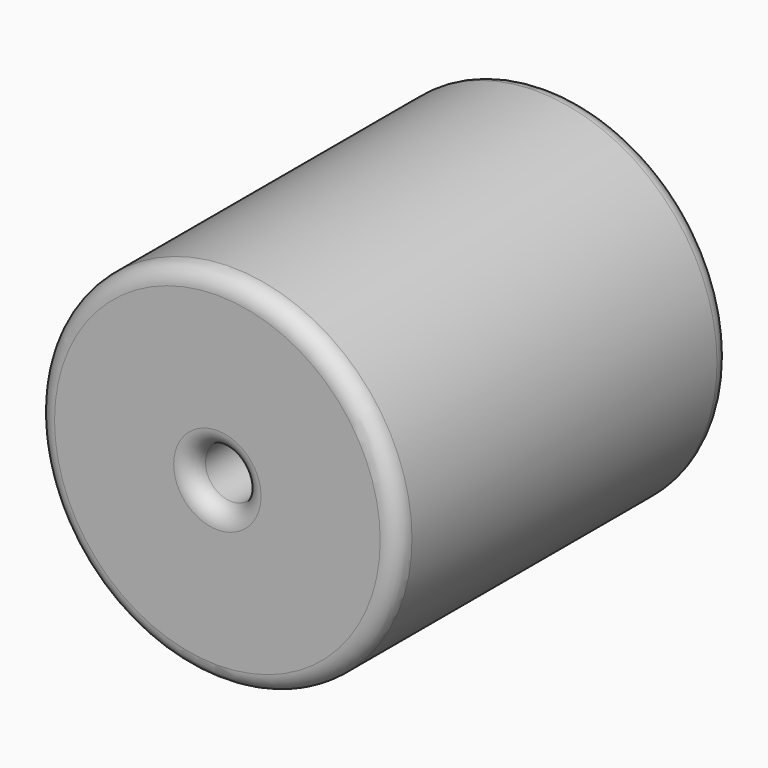
from build123d import *

# Parameters (mm, degrees)
F0_R     = 51.9492240189
F1_DEPTH = 25.4
F2_DEPTH = 94.488
F5_D     = 14.986
F6_R     = 5.08


with BuildPart() as f1:
    # F0 (on Front) → F1 (new body)
    with BuildSketch(Plane.XZ):
        Circle(F0_R)
    extrude(amount=F1_DEPTH)

    # F2 (add): a face of the model
    f2_faces = [f1.faces().sort_by_distance(p)[0] for p in [
        (0, -25.4, 0),
    ]]
    extrude(f2_faces, amount=F2_DEPTH)

    # F5 (through all)
    with Locations(Plane.XZ.offset(119.888)):
        with Locations((0, 0)):
            Hole(F5_D / 2)

    # F6
    f6_edges = [f1.edges().sort_by_distance(p)[0] for p in [
        (-51.949224, -119.888, 0),
        (-51.949224, 0, 0),
        (-7.493, 0, 0),
        (-7.493, -119.888, 0),
    ]]
    fillet(f6_edges, radius=F6_R)


solid = f1.part
